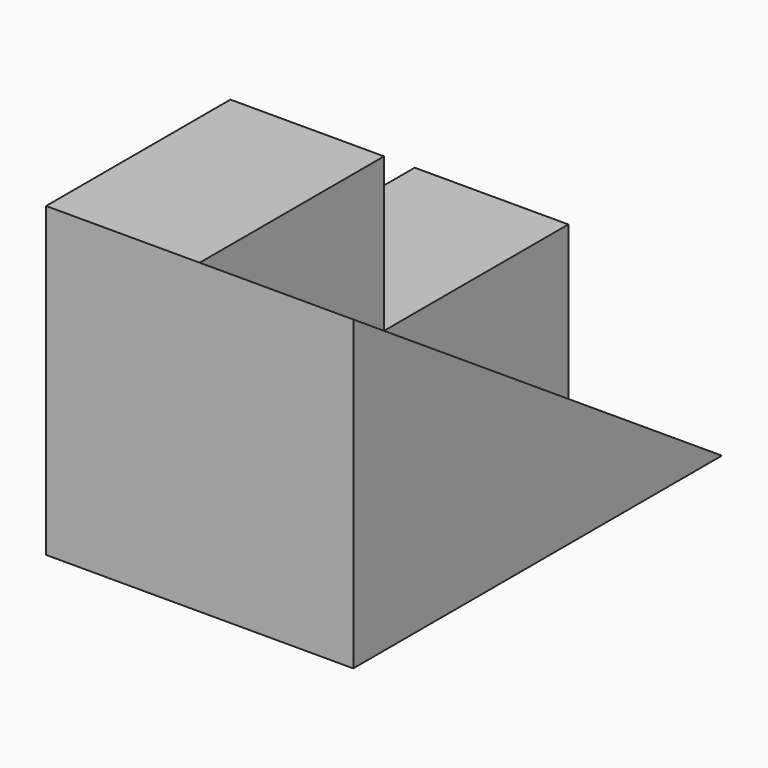
from build123d import *

# Parameters (mm, degrees)
F0_W     = 38.1
F0_H     = 25.4
F1_DEPTH = 12.7
F2_SIZE2 = 25.39999
F2_SIZE  = 38.09999
F4_DEPTH = 12.7


# Not quite as in the source:
# - a fillet or chamfer is up to 0.001 mm smaller than in the source, because OpenCascade refuses the exact size


with BuildPart() as f1:
    # F0 (on Right) → F1 (new body)
    with BuildSketch(Plane.YZ):
        with Locations((-19.05, 12.7)):
            Rectangle(F0_W, F0_H)
    extrude(amount=F1_DEPTH)

    # F2 (size 38.1 and 25.4 in the source; OpenCascade refuses exactly that, so slightly less here)
    f2_edges = [f1.edges().sort_by_distance(p)[0] for p in [
        (6.35, 0, 25.4),
    ]]
    f2_side = f1.faces().sort_by_distance((6.35, -19.05, 25.4))[0]
    chamfer(f2_edges, length=F2_SIZE, length2=F2_SIZE2, reference=f2_side)

    # F3 (on Right) → F4 (join)
    with BuildSketch(Plane.YZ):
        Polygon((-38.1, 0), (0, 0), (0, 12.7), (-19.05, 12.7), (-19.05, 25.4), (-38.1, 25.4), align=None)
    extrude(amount=-F4_DEPTH)


solid = f1.part
